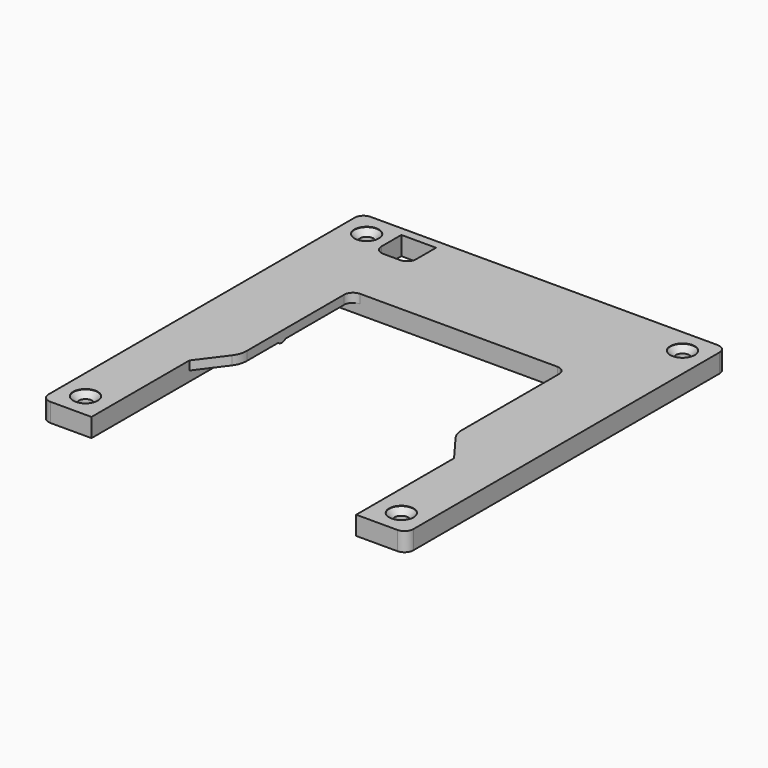
from build123d import *

# Parameters (mm, degrees)
F1_DEPTH      = 2
F3_DEPTH      = 2.2
F5_DEPTH      = 25
F6_R          = 1.5
F7_DEPTH      = 4.2
F8_R          = 2.75
F9_DEPTH      = 1.6
F10_S5_R      = 1.5
F10_T6_DEPTH  = 5
F10_S11_R     = 1.5
F10_T12_DEPTH = 5
F10_S17_R     = 1.5
F10_T18_DEPTH = 5
F10_S23_R     = 1.5
F10_T24_DEPTH = 5
F11_W         = 5.6
F11_H         = 2
F12_DEPTH     = 0.4
F13_T1_DEPTH  = 8.0494897428
F13_T3_DEPTH  = 8.0494897428


# Not quite as in the source:
# - a fillet or chamfer that OpenCascade refuses, or shapes differently, is made with other operations: its cross-section is extruded or revolved along the edge and cut away or added


with BuildPart() as f1:
    # F0 (on Top) → F1 (new body)
    with BuildSketch(Plane.XY):
        with BuildLine():
            Line((80, 0), (2, 0))
            ThreePointArc((2, 0), (0.5857864376, -0.5857864376), (0, -2))
            Line((0, -2), (0, -88))
            ThreePointArc((0, -88), (0.5857864376, -89.4142135624), (2, -90))
            Line((2, -90), (11.25, -90))
            Line((11.25, -90), (11.25, -62.5))
            Line((11.25, -62.5), (15.8564011104, -56.3307127986))
            ThreePointArc((15.8564011104, -56.3307127986), (16.5951030311, -54.9153368199), (16.85, -53.3392666362))
            Line((16.85, -53.3392666362), (16.85, -26))
            ThreePointArc((16.85, -26), (17.4357864376, -24.5857864376), (18.85, -24))
            Line((18.85, -24), (63.15, -24))
            ThreePointArc((63.15, -24), (64.5642135624, -24.5857864376), (65.15, -26))
            Line((65.15, -26), (65.15, -53.3392666362))
            ThreePointArc((65.15, -53.3392666362), (65.4048969689, -54.9153368199), (66.1435988896, -56.3307127986))
            Line((66.1435988896, -56.3307127986), (70.75, -62.5))
            Line((70.75, -62.5), (70.75, -90))
            Line((70.75, -90), (80, -90))
            ThreePointArc((80, -90), (81.4142135624, -89.4142135624), (82, -88))
            Line((82, -88), (82, -2))
            ThreePointArc((82, -2), (81.4142135624, -0.5857864376), (80, 0))
        make_face()
    extrude(amount=F1_DEPTH)

    # F2 (on face) → F3 (join)
    with BuildSketch(Plane(origin=(0, 0, 0), x_dir=(1, 0, 0), z_dir=(0, 0, -1))):
        with BuildLine():
            ThreePointArc((80, 0), (81.4142135624, 0.5857864376), (82, 2))
            Line((82, 2), (82, 88))
            ThreePointArc((82, 88), (81.4142135624, 89.4142135624), (80, 90))
            Line((80, 90), (70.75, 90))
            Line((70.75, 90), (70.75, 62.5))
            Line((70.75, 62.5), (70.75, 26))
            ThreePointArc((70.75, 26), (70.1642135624, 24.5857864376), (68.75, 24))
            Line((68.75, 24), (65.15, 24))
            Line((65.15, 24), (16.85, 24))
            Line((16.85, 24), (13.25, 24))
            ThreePointArc((13.25, 24), (11.8357864376, 24.5857864376), (11.25, 26))
            Line((11.25, 26), (11.25, 62.5))
            Line((11.25, 62.5), (11.25, 90))
            Line((11.25, 90), (2, 90))
            ThreePointArc((2, 90), (0.5857864376, 89.4142135624), (0, 88))
            Line((0, 88), (0, 2))
            ThreePointArc((0, 2), (0.5857864376, 0.5857864376), (2, 0))
            Line((2, 0), (80, 0))
        make_face()
    extrude(amount=F3_DEPTH)

    # F4 (on face) → F5 (cut)
    with BuildSketch(Plane.XY.offset(2)):
        with BuildLine():
            Line((18.3, -2), (10.5, -2))
            Line((10.5, -2), (10.5, -7.6))
            ThreePointArc((10.5, -7.6), (11.0857864376, -9.0142135624), (12.5, -9.6))
            Line((12.5, -9.6), (16.3, -9.6))
            ThreePointArc((16.3, -9.6), (17.7142135624, -9.0142135624), (18.3, -7.6))
            Line((18.3, -7.6), (18.3, -2))
        make_face()
    extrude(amount=-F5_DEPTH, mode=Mode.SUBTRACT)

    # F6 (on face) → F7 (cut)
    with BuildSketch(Plane.XY.offset(2)):
        with Locations((5.5, -84.5)):
            Circle(F6_R)
        with Locations((76.5, -84.5)):
            Circle(F6_R)
        with Locations((5.5, -5.5)):
            Circle(F6_R)
        with Locations((76.5, -5.5)):
            Circle(F6_R)
    extrude(amount=-F7_DEPTH, mode=Mode.SUBTRACT)

    # F8 (on face) → F9 (cut)
    with BuildSketch(Plane.XY.offset(2)):
        with Locations((5.5, -5.5)):
            Circle(F8_R)
        with Locations((76.5, -5.5)):
            Circle(F8_R)
        with Locations((76.5, -84.5)):
            Circle(F8_R)
        with Locations((5.5, -84.5)):
            Circle(F8_R)
    extrude(amount=-F9_DEPTH, mode=Mode.SUBTRACT)

    # F10: chamfer of 1.5 on 4 edges, made by hand


with BuildPart() as f10_tool2:
    # F10_s3 → F10_t4 (revolve)
    with BuildSketch(Plane.XZ.offset(84.5)):
        Polygon((8.25, 1.9), (6.75, 0.4), (8.25, 0.4), align=None)
    revolve(axis=Axis((5.5, -84.5, 0.4), (0, 0, 1)))

    # F10_s5 → F10_t6 (cut, symmetric)
    with BuildSketch(Plane.XY.offset(1.1)):
        with Locations((5.5, -84.5)):
            Circle(F10_S5_R)
    extrude(amount=F10_T6_DEPTH, both=True, mode=Mode.SUBTRACT)


with BuildPart() as f1_1:
    add(f1.part)

    # F10_t1: union F10_tool2
    add(f10_tool2.part)


with BuildPart() as f10_tool8:
    # F10_s9 → F10_t10 (revolve)
    with BuildSketch(Plane.XZ.offset(84.5)):
        Polygon((79.25, 1.9), (77.75, 0.4), (79.25, 0.4), align=None)
    revolve(axis=Axis((76.5, -84.5, 0.4), (0, 0, 1)))

    # F10_s11 → F10_t12 (cut, symmetric)
    with BuildSketch(Plane.XY.offset(1.1)):
        with Locations((76.5, -84.5)):
            Circle(F10_S11_R)
    extrude(amount=F10_T12_DEPTH, both=True, mode=Mode.SUBTRACT)


with BuildPart() as f1_2:
    add(f1_1.part)

    # F10_t7: union F10_tool8
    add(f10_tool8.part)


with BuildPart() as f10_tool14:
    # F10_s15 → F10_t16 (revolve)
    with BuildSketch(Plane.XZ.offset(5.5)):
        Polygon((8.25, 1.9), (6.75, 0.4), (8.25, 0.4), align=None)
    revolve(axis=Axis((5.5, -5.5, 0.4), (0, 0, 1)))

    # F10_s17 → F10_t18 (cut, symmetric)
    with BuildSketch(Plane.XY.offset(1.1)):
        with Locations((5.5, -5.5)):
            Circle(F10_S17_R)
    extrude(amount=F10_T18_DEPTH, both=True, mode=Mode.SUBTRACT)


with BuildPart() as f1_3:
    add(f1_2.part)

    # F10_t13: union F10_tool14
    add(f10_tool14.part)


with BuildPart() as f10_tool20:
    # F10_s21 → F10_t22 (revolve)
    with BuildSketch(Plane.XZ.offset(5.5)):
        Polygon((79.25, 1.9), (77.75, 0.4), (79.25, 0.4), align=None)
    revolve(axis=Axis((76.5, -5.5, 0.4), (0, 0, 1)))

    # F10_s23 → F10_t24 (cut, symmetric)
    with BuildSketch(Plane.XY.offset(1.1)):
        with Locations((76.5, -5.5)):
            Circle(F10_S23_R)
    extrude(amount=F10_T24_DEPTH, both=True, mode=Mode.SUBTRACT)


with BuildPart() as f1_4:
    add(f1_3.part)

    # F10_t19: union F10_tool20
    add(f10_tool20.part)

    # F11 (on face) → F12 (join)
    with BuildSketch(Plane(origin=(0, 0, 0), x_dir=(1, 0, 0), z_dir=(0, 0, -1))):
        with Locations((14.05, 43.5)):
            Rectangle(F11_W, F11_H)
        with Locations((67.95, 43.5)):
            Rectangle(F11_W, F11_H)
    extrude(amount=F12_DEPTH)

    # F13: fillet of radius 1.4 on 4 edges, made by hand

    # F13_s2 → F13_t1 (cut)
    with BuildSketch(Plane.YZ.offset(11.25)):
        with BuildLine():
            ThreePointArc((-42.5, 0), (-42.9506456349, -0.2961481397), (-43.4797958971, -0.4))
            Line((-43.4797958971, -0.4), (-42.5, -0.4))
            Line((-42.5, -0.4), (-42.5, 0))
        make_face()
        with BuildLine():
            ThreePointArc((-43.5202041029, -0.4), (-44.0493543651, -0.2961481397), (-44.5, 0))
            Line((-44.5, 0), (-44.5, -0.4))
            Line((-44.5, -0.4), (-43.5202041029, -0.4))
        make_face()
    extrude(amount=F13_T1_DEPTH, mode=Mode.SUBTRACT)

    # F13_s4 → F13_t3 (cut)
    with BuildSketch(Plane.YZ.offset(62.7005102572)):
        with BuildLine():
            ThreePointArc((-43.4797958971, -0.4), (-42.9506456349, -0.2961481397), (-42.5, 0))
            Line((-42.5, 0), (-42.5, -0.4))
            Line((-42.5, -0.4), (-43.4797958971, -0.4))
        make_face()
        with BuildLine():
            ThreePointArc((-44.5, 0), (-44.0493543651, -0.2961481397), (-43.5202041029, -0.4))
            Line((-43.5202041029, -0.4), (-44.5, -0.4))
            Line((-44.5, -0.4), (-44.5, 0))
        make_face()
    extrude(amount=F13_T3_DEPTH, mode=Mode.SUBTRACT)


solid = f1_4.part
